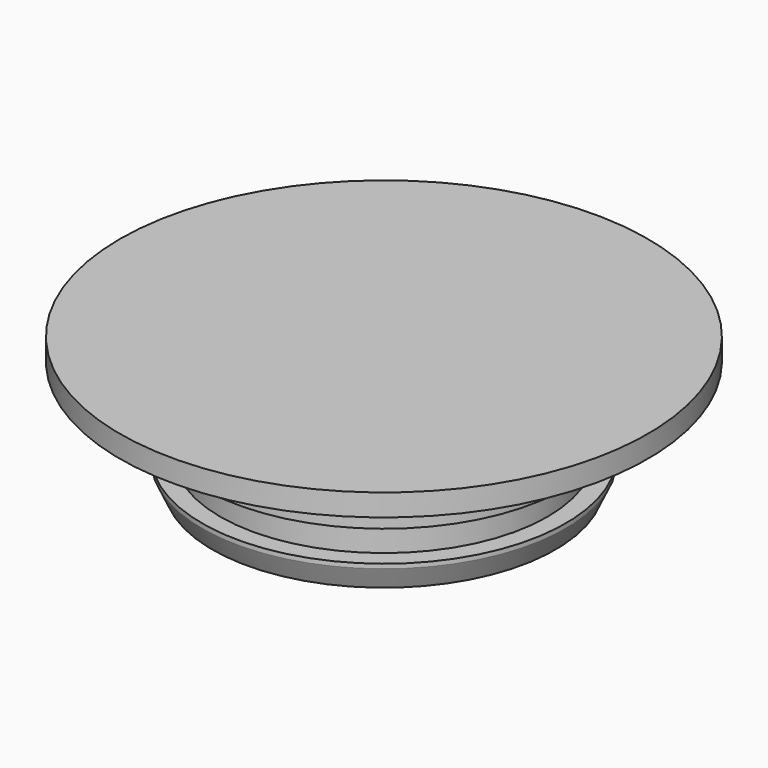
from build123d import *


# Not quite as in the source:
# - a feature names something its author has since deleted; it is built from what else it names


with BuildPart() as f1:
    # F0 (on Front) → F1 (revolve)
    with BuildSketch(Plane.XZ):
        Polygon((0, -12.5), (0, -12), (0, 0), (0, 5), (-60, 5), (-60, 0), (-47.5, 0), (-41.3, 0), (-41.3, -12), (-37.2, -12), (-37.2, -19), (-41.3, -19), (-41.3, -20), (-39, -25), (0, -25), align=None)
    revolve(axis=Axis((0, 0, -12.5), (0, 0, -1)))


solid = f1.part
